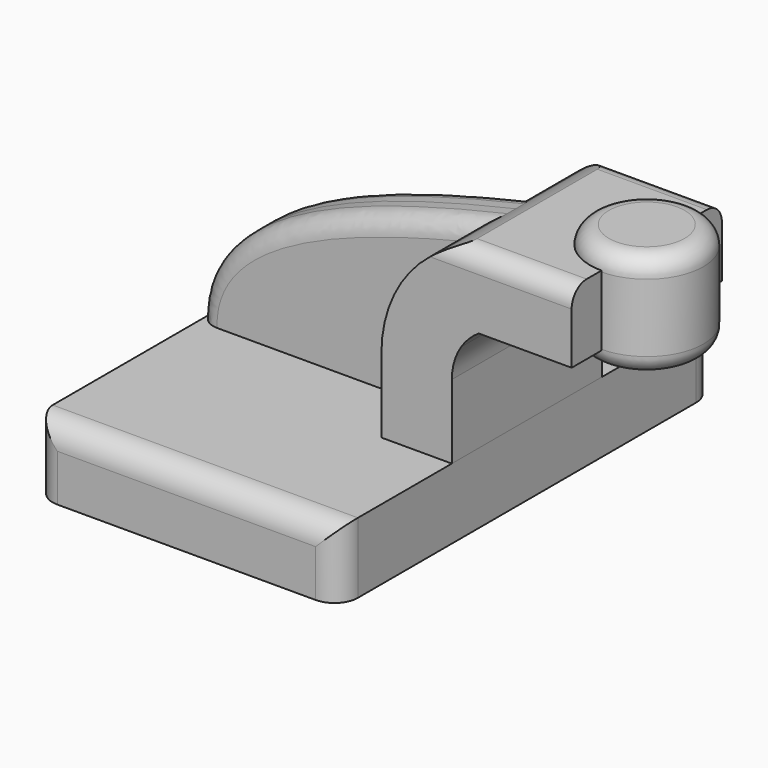
from build123d import *

# Parameters (mm, degrees)
F1_DEPTH    = 63.5
F2_DEPTH    = 7.9375
F3_DEPTH    = 25.4
F5_R        = 6.35
F6_T1_DEPTH = 55.0007445182
F6_2_F1_R   = 5.08
F6_2_F2_R   = 5.08


# Not quite as in the source:
# - a fillet or chamfer that OpenCascade refuses, or shapes differently, is made with other operations: its cross-section is extruded or revolved along the edge and cut away or added


with BuildPart() as f1:
    # F0 (on Front) → F1 (new body, symmetric)
    with BuildSketch(Plane.XZ):
        Polygon((-41.275, 9.525), (-41.275, -9.525), (41.275, -9.525), (41.275, 9.525), (22.225, 9.525), align=None)
    extrude(amount=F1_DEPTH, both=True)

    # F5
    f5_edges = [f1.edges().sort_by_distance(p)[0] for p in [
        (-41.275, -63.5, 0),
        (41.275, -63.5, 0),
        (41.275, 63.5, 0),
        (-41.275, 63.5, 0),
        (0, 63.5, 9.525),
        (0, -63.5, 9.525),
    ]]
    fillet(f5_edges, radius=F5_R)


with BuildPart() as f2:
    # F0 (on Front) → F2 (new body, symmetric)
    with BuildSketch(Plane.XZ):
        with BuildLine():
            add(Edge.make_bspline(
                [(-41.275, 9.525), (-41.9218663516, 37.3261011822), (0, 50.0849671662), (38.1976362328, 58.8767082382)],
                knots=[0, 0, 0, 0, 93.5494041446, 93.5494041446, 93.5494041446, 93.5494041446], degree=3))
            Line((-41.275, 9.525), (22.225, 9.525))
            Line((22.225, 9.525), (22.225, 29.5413450627))
            ThreePointArc((22.225, 29.5413450627), (26.4769912662, 46.2423079157), (38.1976362328, 58.8767082382))
        make_face()
    extrude(amount=F2_DEPTH, both=True)

    # F6#2: fillet of radius 5.08 on 2 edges, made by hand

    # F6_2_f1
    f6_2_f1_edges = [f2.edges().sort_by_distance(p)[0] for p in [
        (-16.1053703527, 7.9375, 41.3293641604),
    ]]
    fillet(f6_2_f1_edges, radius=F6_2_F1_R)

    # F6_2_f2
    f6_2_f2_edges = [f2.edges().sort_by_distance(p)[0] for p in [
        (-16.1053703527, -7.9375, 41.3293641604),
    ]]
    fillet(f6_2_f2_edges, radius=F6_2_F2_R)


with BuildPart() as f3:
    # F0 (on Front) → F3 (new body, symmetric)
    with BuildSketch(Plane.XZ):
        with BuildLine():
            Line((22.225, 9.525), (41.275, 9.525))
            Line((41.275, 9.525), (41.275, 29.5413450627))
            ThreePointArc((41.275, 29.5413450627), (41.9140357405, 34.0001585915), (43.7796951918, 38.1))
            Line((43.7796951918, 38.1), (38.1976362328, 38.1))
            Line((38.1976362328, 38.1), (38.1976362328, 58.8767082382))
            ThreePointArc((38.1976362328, 58.8767082382), (26.4769912662, 46.2423079157), (22.225, 29.5413450627))
            Line((22.225, 29.5413450627), (22.225, 9.525))
        make_face()
        with BuildLine():
            ThreePointArc((44.0717140113, 61.9252), (41.0623041907, 60.5404042186), (38.1976362328, 58.8767082382))
            Line((38.1976362328, 58.8767082382), (38.1976362328, 38.1))
            Line((38.1976362328, 38.1), (43.7796951918, 38.1))
            ThreePointArc((43.7796951918, 38.1), (45.9008806945, 40.7428154953), (48.5346684619, 42.8752))
            Line((48.5346684619, 42.8752), (73.6724585295, 42.8752))
            Line((73.6724585295, 42.8752), (73.6724585295, 61.9252))
            Line((73.6724585295, 61.9252), (44.0717140113, 61.9252))
        make_face()
    extrude(amount=F3_DEPTH, both=True)

    # F0 (on Front) → F4 (revolve)
    with BuildSketch(Plane.XZ):
        Polygon((88.9976362328, 66.675), (73.6724585295, 66.675), (73.6724585295, 61.9252), (73.6724585295, 42.8752), (73.6724585295, 38.1), (88.9976362328, 38.1), align=None)
    revolve(axis=Axis((73.6724585295, 0, 52.3875), (0, 0, 1)))

    # F6: fillet of radius 5.08 on 4 edges, made by hand

    # F6_s2 → F6_t1 (cut)
    with BuildSketch(Plane.YZ.offset(31.3717140113)):
        with BuildLine():
            ThreePointArc((-25.4, 56.8452), (-23.9121024484, 60.4373024484), (-20.32, 61.9252))
            Line((-20.32, 61.9252), (-25.4, 61.9252))
            Line((-25.4, 61.9252), (-25.4, 56.8452))
        make_face()
        with BuildLine():
            ThreePointArc((25.4, 56.8452), (23.9121024484, 60.4373024484), (20.32, 61.9252))
            Line((20.32, 61.9252), (25.4, 61.9252))
            Line((25.4, 61.9252), (25.4, 56.8452))
        make_face()
    extrude(amount=F6_T1_DEPTH, mode=Mode.SUBTRACT)


with BuildPart() as f6_tool4:
    # F6_s5 → F6_t6 (revolve)
    with BuildSketch(Plane.XZ):
        with BuildLine():
            ThreePointArc((88.9976362328, 43.18), (87.5097386812, 39.5878975516), (83.9176362328, 38.1))
            Line((83.9176362328, 38.1), (88.9976362328, 38.1))
            Line((88.9976362328, 38.1), (88.9976362328, 43.18))
        make_face()
    revolve(axis=Axis((73.6724585295, 0, 38.1), (0, 0, 1)))

    split(bisect_by=Plane.XY.offset(42.8752), keep=Keep.TOP)

    split(bisect_by=Plane.YZ.offset(73.6724585295), keep=Keep.TOP)


with BuildPart() as f3_1:
    add(f3.part)

    # F6_t3: cut F6_tool4
    add(f6_tool4.part, mode=Mode.SUBTRACT)


with BuildPart() as f6_tool10:
    # F6_s11 → F6_t12 (revolve)
    with BuildSketch(Plane.XZ):
        with BuildLine():
            ThreePointArc((88.9976362328, 43.18), (87.5097386812, 39.5878975516), (83.9176362328, 38.1))
            Line((83.9176362328, 38.1), (88.9976362328, 38.1))
            Line((88.9976362328, 38.1), (88.9976362328, 43.18))
        make_face()
    revolve(axis=Axis((73.6724585295, 0, 38.1), (0, 0, 1)))

    split(bisect_by=Plane.XY.offset(42.8752), keep=Keep.BOTTOM)

    split(bisect_by=Plane.YZ.offset(73.6724585295), keep=Keep.TOP)


with BuildPart() as f3_2:
    add(f3_1.part)

    # F6_t9: cut F6_tool10
    add(f6_tool10.part, mode=Mode.SUBTRACT)


with BuildPart() as f6_tool16:
    # F6_s17 → F6_t18 (revolve)
    with BuildSketch(Plane.XZ):
        with BuildLine():
            ThreePointArc((88.9976362328, 43.18), (87.5097386812, 39.5878975516), (83.9176362328, 38.1))
            Line((83.9176362328, 38.1), (88.9976362328, 38.1))
            Line((88.9976362328, 38.1), (88.9976362328, 43.18))
        make_face()
    revolve(axis=Axis((73.6724585295, 0, 38.1), (0, 0, 1)))

    split(bisect_by=Plane.XY.offset(42.8752), keep=Keep.BOTTOM)

    split(bisect_by=Plane.YZ.offset(73.6724585295), keep=Keep.BOTTOM)


with BuildPart() as f3_3:
    add(f3_2.part)

    # F6_t15: cut F6_tool16
    add(f6_tool16.part, mode=Mode.SUBTRACT)


with BuildPart() as f6_tool22:
    # F6_s23 → F6_t24 (revolve)
    with BuildSketch(Plane.XZ):
        with BuildLine():
            ThreePointArc((88.9976362328, 61.595), (87.5097386812, 65.1871024484), (83.9176362328, 66.675))
            Line((83.9176362328, 66.675), (88.9976362328, 66.675))
            Line((88.9976362328, 66.675), (88.9976362328, 61.595))
        make_face()
    revolve(axis=Axis((73.6724585295, 0, 66.675), (0, 0, 1)))

    split(bisect_by=Plane.YZ.offset(73.6724585295), keep=Keep.TOP)

    split(bisect_by=Plane.XY.offset(61.9252), keep=Keep.BOTTOM)


with BuildPart() as f3_4:
    add(f3_3.part)

    # F6_t21: cut F6_tool22
    add(f6_tool22.part, mode=Mode.SUBTRACT)


with BuildPart() as f6_tool28:
    # F6_s29 → F6_t30 (revolve)
    with BuildSketch(Plane.XZ):
        with BuildLine():
            ThreePointArc((88.9976362328, 61.595), (87.5097386812, 65.1871024484), (83.9176362328, 66.675))
            Line((83.9176362328, 66.675), (88.9976362328, 66.675))
            Line((88.9976362328, 66.675), (88.9976362328, 61.595))
        make_face()
    revolve(axis=Axis((73.6724585295, 0, 66.675), (0, 0, 1)))

    split(bisect_by=Plane.YZ.offset(73.6724585295), keep=Keep.TOP)

    split(bisect_by=Plane.XY.offset(61.9252), keep=Keep.TOP)


with BuildPart() as f3_5:
    add(f3_4.part)

    # F6_t27: cut F6_tool28
    add(f6_tool28.part, mode=Mode.SUBTRACT)


with BuildPart() as f6_tool34:
    # F6_s35 → F6_t36 (revolve)
    with BuildSketch(Plane.XZ):
        with BuildLine():
            ThreePointArc((88.9976362328, 61.595), (87.5097386812, 65.1871024484), (83.9176362328, 66.675))
            Line((83.9176362328, 66.675), (88.9976362328, 66.675))
            Line((88.9976362328, 66.675), (88.9976362328, 61.595))
        make_face()
    revolve(axis=Axis((73.6724585295, 0, 66.675), (0, 0, 1)))

    split(bisect_by=Plane.YZ.offset(73.6724585295), keep=Keep.BOTTOM)

    split(bisect_by=Plane.XY.offset(61.9252), keep=Keep.TOP)


with BuildPart() as f3_6:
    add(f3_5.part)

    # F6_t33: cut F6_tool34
    add(f6_tool34.part, mode=Mode.SUBTRACT)


solid = Compound([f1.part, f2.part, f3_6.part])
